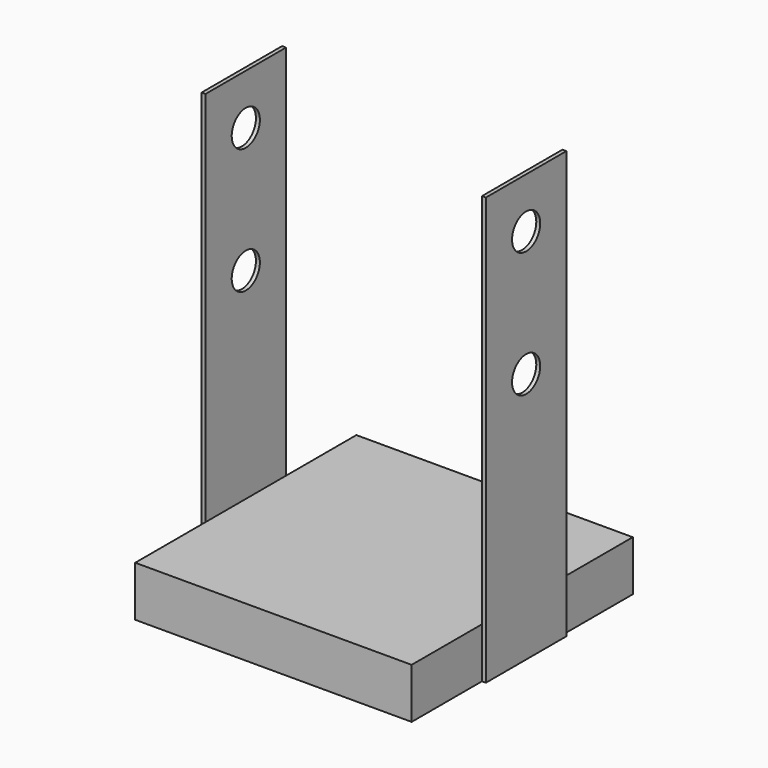
from build123d import *

# Parameters (mm, degrees)
F0_W     = 134.112
F0_H     = 134.112
F1_DEPTH = 25.4
F2_DEPTH = 2.794
F0_W_2   = 1.9812
F0_H_2   = 50.8
F3_DEPTH = 190.5
F4_DEPTH = 25.4
F5_R     = 8.89
F6_DEPTH = 143.6634


# Not quite as in the source:
# - a feature of the source that left no trace in its solid (it failed there, or was rolled back) is left out


with BuildPart() as f1:
    # F0 (on Top) → F1 (new body)
    with BuildSketch(Plane.XY):
        Polygon((0, 44.45), (0, 0), (139.7, 0), (139.7, 44.45), (139.7, 95.25), (139.7, 139.7), (0, 139.7), (0, 95.25), align=None)
        with Locations((69.85, 69.85)):
            Rectangle(F0_W, F0_H, mode=Mode.SUBTRACT)
    extrude(amount=-F1_DEPTH)

    # F0 (on Top) → F2 (join)
    with BuildSketch(Plane.XY):
        with Locations((69.85, 69.85)):
            Rectangle(F0_W, F0_H)
    extrude(amount=-F2_DEPTH)

    # F0 (on Top) → F3 (join)
    with BuildSketch(Plane.XY):
        with Locations((-0.9906, 69.85)):
            Rectangle(F0_W_2, F0_H_2)
        with Locations((140.6906, 69.85)):
            Rectangle(F0_W_2, F0_H_2)
    extrude(amount=F3_DEPTH)

    # F0 (on Top) → F4 (join)
    with BuildSketch(Plane.XY):
        with Locations((-0.9906, 69.85)):
            Rectangle(F0_W_2, F0_H_2)
        with Locations((140.6906, 69.85)):
            Rectangle(F0_W_2, F0_H_2)
    extrude(amount=-F4_DEPTH)

    # F5 (on face) → F6 (cut, through all)
    with BuildSketch(Plane.YZ.offset(141.6812)):
        with Locations((69.85, 165.1)):
            Circle(F5_R)
        with Locations((69.85, 101.6)):
            Circle(F5_R)
    extrude(amount=-F6_DEPTH, mode=Mode.SUBTRACT)


solid = f1.part
